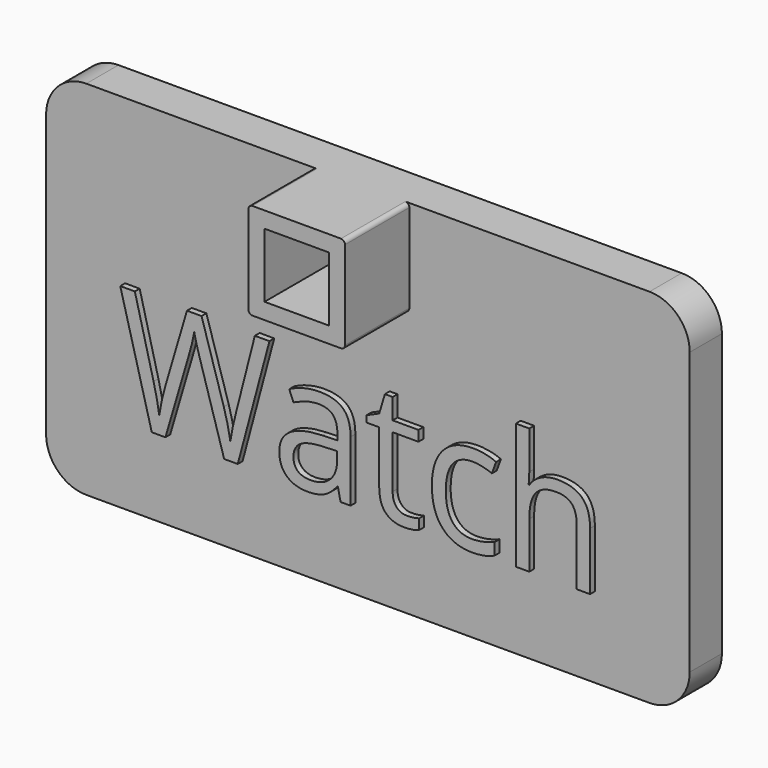
from build123d import *

# Parameters (mm, degrees)
F0_W         = 80
F0_H         = 45
F1_DEPTH     = 5
F2_R         = 5
F3_W         = 12
F3_H         = 12
F4_DEPTH     = 10
F5_W         = 8
F5_H         = 8
F6_DEPTH     = 10
F7_R         = 0.5
F8_TEXT_SIZE = 20.625201418
F9_DEPTH     = 0.75
F10_R        = 5
F11_DEPTH    = 1.5


# Not quite as in the source:
# - Text() gives the source's letters only with a copy of the font that has no kerning and outlines rounded to 1/6400 em; it was checked with that copy


with BuildPart() as f1:
    # F0 (on Front) → F1 (new body)
    with BuildSketch(Plane.XZ):
        Rectangle(F0_W, F0_H)
    extrude(amount=F1_DEPTH)

    # F2
    f2_edges = [f1.edges().sort_by_distance(p)[0] for p in [
        (40, -2.5, 22.5),
        (40, -2.5, -22.5),
        (-40, -2.5, -22.5),
        (-40, -2.5, 22.5),
    ]]
    fillet(f2_edges, radius=F2_R)

    # F3 (on face) → F4 (join)
    with BuildSketch(Plane.XZ.offset(5)):
        with Locations((-0.8478262983, 16.5)):
            Rectangle(F3_W, F3_H)
    extrude(amount=F4_DEPTH)

    # F5 (on face) → F6 (cut)
    with BuildSketch(Plane.XZ.offset(15)):
        with Locations((-0.8478262983, 16.5)):
            Rectangle(F5_W, F5_H)
    extrude(amount=-F6_DEPTH, mode=Mode.SUBTRACT)

    # F7
    f7_edges = [f1.edges().sort_by_distance(p)[0] for p in [
        (5.152174, -10, 10.5),
        (-6.847826, -10, 10.5),
        (-6.847826, -10, 22.5),
        (5.152174, -10, 22.5),
    ]]
    fillet(f7_edges, radius=F7_R)

    # F8 (on face) → F9 (join)
    with BuildSketch(Plane.XZ.offset(5)):
        with Locations((-30.45220121, -12.5)):
            Text('Watch', F8_TEXT_SIZE, font='Open Sans', text_align=(TextAlign.LEFT, TextAlign.BOTTOM))
    extrude(amount=F9_DEPTH)

    # F10 (on face) → F11 (cut)
    with BuildSketch(Plane(origin=(0, 0, 0), x_dir=(-1, 0, 0), z_dir=(0, 1, 0))):
        with Locations((-32, 14.5)):
            Circle(F10_R)
        with Locations((32, 14.5)):
            Circle(F10_R)
        with Locations((32, -14.5)):
            Circle(F10_R)
        with Locations((-32, -14.5)):
            Circle(F10_R)
    extrude(amount=-F11_DEPTH, mode=Mode.SUBTRACT)


solid = f1.part
